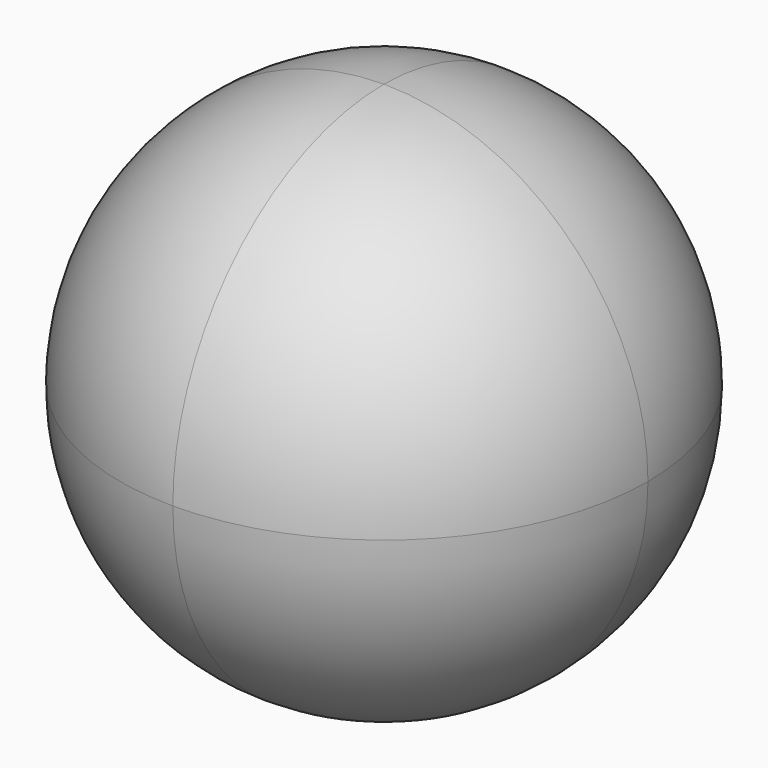
from build123d import *

# Parameters (mm, degrees)
F0_W     = 35.5
F0_H     = 35.5
F1_DEPTH = 35.5
F2_R     = 17.74999
F3_DEPTH = 1.5


# Not quite as in the source:
# - a fillet or chamfer is up to 0.001 mm smaller than in the source, because OpenCascade refuses the exact size


with BuildPart() as f1:
    # F0 (on Top) → F1 (new body)
    with BuildSketch(Plane.XY):
        Rectangle(F0_W, F0_H)
    extrude(amount=F1_DEPTH)

    # F2 (radius 17.75 in the source; OpenCascade refuses exactly that, so slightly less here)
    f2_edges = [f1.edges().sort_by_distance(p)[0] for p in [
        (0, 17.75, 35.5),
        (-17.75, 0, 35.5),
        (0, -17.75, 35.5),
        (17.75, 0, 35.5),
        (17.75, 17.75, 17.75),
        (-17.75, 17.75, 17.75),
        (0, 17.75, 0),
        (17.75, -17.75, 17.75),
        (17.75, 0, 0),
        (-17.75, 0, 0),
        (0, -17.75, 0),
        (-17.75, -17.75, 17.75),
    ]]
    fillet(f2_edges, radius=F2_R)


with BuildPart() as f3:
    # F0 (on Top) → F3 (new body, symmetric)
    with BuildSketch(Plane.XY):
        Rectangle(F0_W, F0_H)
    extrude(amount=F3_DEPTH, both=True)


with BuildPart() as f1_1:
    add(f1.part)

    # F4: cut F3
    add(f3.part, mode=Mode.SUBTRACT)


solid = f1_1.part
